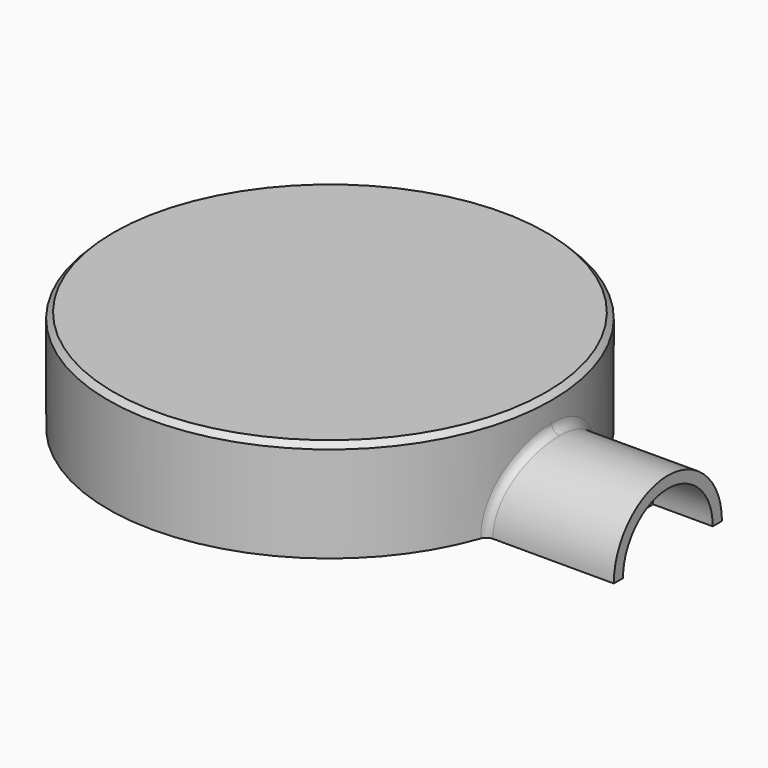
from build123d import *
from build123d import SkipClean  # not in build123d's __all__

# Parameters (mm, degrees)
F0_R      = 16.4
F1_DEPTH  = 15
F2_R      = 15.2
F3_DEPTH  = 2
F4_R      = 11
F5_DEPTH  = 25
F6_R      = 15.2
F7_DEPTH  = 10.4
F8_R      = 15.5
F9_DEPTH  = 6
F10_R     = 6.2
F11_DEPTH = 5
F13_DEPTH = 5
F15_START = 15.2
F14_R     = 5
F15_DEPTH = 9.8
F16_R     = 0.6
F17_SIZE  = 0.4
F18_R     = 4.15
F19_DEPTH = 4.4
F21_R     = 45.33445
F22_DEPTH = 25


with BuildPart() as f1:
    # F0 (on Top) → F1 (new body)
    with BuildSketch(Plane.XY):
        Circle(F0_R)
    extrude(amount=F1_DEPTH)

    # F2 (on face) → F3 (cut)
    with BuildSketch(Plane(origin=(0, 0, 0), x_dir=(1, 0, 0), z_dir=(0, 0, -1))):
        Circle(F2_R)
    extrude(amount=-F3_DEPTH, mode=Mode.SUBTRACT)

    # F4 (on face) → F5 (cut)
    with BuildSketch(Plane(origin=(0, 0, 2), x_dir=(1, 0, 0), z_dir=(0, 0, -1))):
        Circle(F4_R)
    extrude(amount=-F5_DEPTH, mode=Mode.SUBTRACT)

    # F6 (on face) → F7 (cut)
    with BuildSketch(Plane.XY.offset(15)):
        Circle(F6_R)
    extrude(amount=-F7_DEPTH, mode=Mode.SUBTRACT)

    # F8 (on face) → F9 (join)
    with BuildSketch(Plane.XY.offset(15)):
        Circle(F8_R)
    extrude(amount=-F9_DEPTH)

    # F10 (on face) → F11 (cut)
    with BuildSketch(Plane(origin=(0, 0, 9), x_dir=(1, 0, 0), z_dir=(0, 0, -1))):
        Circle(F10_R)
    extrude(amount=-F11_DEPTH, mode=Mode.SUBTRACT)

    # F12 (on face) → F13 (cut)
    with BuildSketch(Plane(origin=(0, 0, 2), x_dir=(1, 0, 0), z_dir=(0, 0, -1))):
        with BuildLine():
            Line((1.5, 10.897247), (1.5, 15.125806))
            ThreePointArc((1.5, 15.125806), (0, 15.2), (-1.5, 15.125806))
            Line((-1.5, 15.125806), (-1.5, 10.897247))
            ThreePointArc((-1.5, 10.897247), (0, 11), (1.5, 10.897247))
        make_face()
        with BuildLine():
            Line((-1.5, -10.897247), (-1.5, -15.125806))
            ThreePointArc((-1.5, -15.125806), (0, -15.2), (1.5, -15.125806))
            Line((1.5, -15.125806), (1.5, -10.897247))
            ThreePointArc((1.5, -10.897247), (0, -11), (-1.5, -10.897247))
        make_face()
    with SkipClean():  # cleaning this boolean's faces spoils the solid; the shape is the same uncleaned
        extrude(amount=-F13_DEPTH, mode=Mode.SUBTRACT)

    # F14 (on Right) → F15 (join)
    with BuildSketch(Plane.YZ.offset(F15_START)):
        with Locations((0, 7.5)):
            Circle(F14_R)
    with SkipClean():  # cleaning this boolean's faces spoils the solid; the shape is the same uncleaned
        extrude(amount=F15_DEPTH)

    # F16
    f16_edges = [f1.edges().sort_by_distance(p)[0] for p in [
        (15.619219, -5, 7.5),
        (16.014293, 3.535878, 11.03519),
        (16.014293, 3.535877, 3.96481),
    ]]
    fillet(f16_edges, radius=F16_R)

    # F17
    f17_edges = [f1.edges().sort_by_distance(p)[0] for p in [
        (-16.4, 0, 0),
        (-16.4, 0, 15),
    ]]
    chamfer(f17_edges, length=F17_SIZE)

    # F18 (on face) → F19 (cut)
    with BuildSketch(Plane.YZ.offset(25)):
        with Locations((0, 7.5)):
            Circle(F18_R)
    with SkipClean():  # cleaning this boolean's faces spoils the solid; the shape is the same uncleaned
        extrude(amount=-F19_DEPTH, mode=Mode.SUBTRACT)

    # F21 (on offset) → F22 (cut)
    with BuildSketch(Plane.XY.offset(7.5)):
        Circle(F21_R)
    extrude(amount=-F22_DEPTH, mode=Mode.SUBTRACT)


solid = f1.part
